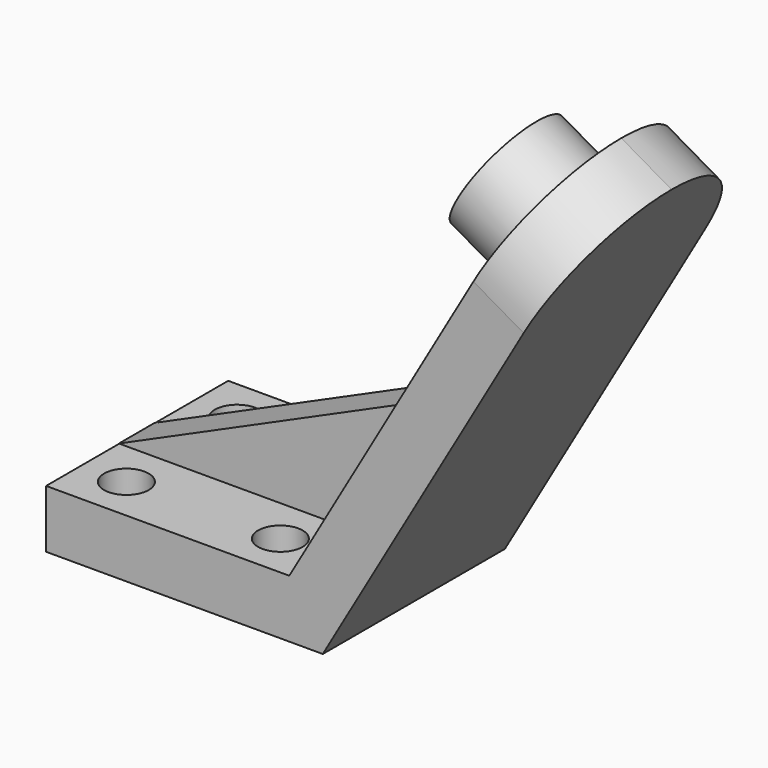
from build123d import *

# Parameters (mm, degrees)
F1_DEPTH = 259.08
F2_R     = 68.58
F2_R_2   = 46.99
F3_DEPTH = 76.2
F4_R     = 129.53999
F7_DEPTH = 25.4
F8_R     = 25.4
F9_DEPTH = 76.2


# Not quite as in the source:
# - a fillet or chamfer is up to 0.001 mm smaller than in the source, because OpenCascade refuses the exact size


with BuildPart() as f1:
    # F0 (on Front) → F1 (new body)
    with BuildSketch(Plane.XZ):
        Polygon((39.5514294499, 0), (-237.3085705501, 0), (-237.3085705501, -66.04), (77.6796412272, -66.04), (371.0496412272, 442.0917454165), (313.8573235613, 475.1117454165), align=None)
    extrude(amount=F1_DEPTH)

    # F2 (on face) → F3 (join)
    with BuildSketch(Plane(origin=(29.6635720874, 0, -17.1262713298), x_dir=(0, -1, 0), z_dir=(-0.8660254038, 0, 0.5))):
        with Locations((129.54, 438.8475029477)):
            Circle(F2_R)
        with Locations((129.54, 438.8475029477)):
            Circle(F2_R_2, mode=Mode.SUBTRACT)
    extrude(amount=F3_DEPTH)

    # F4 (radius 129.54 in the source; OpenCascade refuses exactly that, so slightly less here)
    f4_edges = [f1.edges().sort_by_distance(p)[0] for p in [
        (342.453482, -259.08, 458.601745),
        (342.453482, 0, 458.601745),
    ]]
    fillet(f4_edges, radius=F4_R)

    # F6 (on offset) → F7 (join, symmetric)
    with BuildSketch(Plane.XZ.offset(129.54)):
        Polygon((136.0714294499, 167.1775439465), (-237.7703315524, 0), (39.5514294499, 0), align=None)
    extrude(amount=F7_DEPTH, both=True)

    # F8 (on face) → F9 (cut)
    with BuildSketch(Plane.XY):
        with Locations((-186.5085705501, -50.8)):
            Circle(F8_R)
        with Locations((-186.5085705501, -208.28)):
            Circle(F8_R)
        with Locations((-11.2485705501, -50.8)):
            Circle(F8_R)
        with Locations((-11.2485705501, -208.28)):
            Circle(F8_R)
    extrude(amount=-F9_DEPTH, mode=Mode.SUBTRACT)


solid = f1.part
